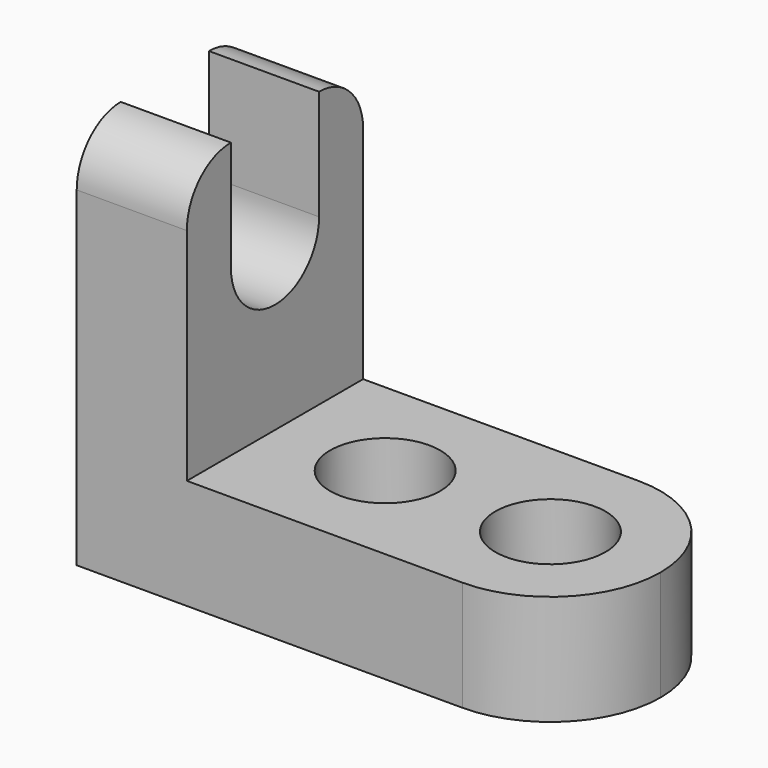
from build123d import *

# Parameters (mm, degrees)
F0_W      = 57.15
F0_H      = 12.7
F1_DEPTH  = 25.4
F2_W      = 12.7
F2_H      = 25.4
F3_DEPTH  = 31.75
F4_R      = 6.35
F5_DEPTH  = 12.701
F7_DEPTH  = 25.4
F9_DEPTH  = 12.701
F10_DEPTH = 25.4
F12_DEPTH = 12.701


# Not quite as in the source:
# - ends of sketch curves that miss each other by under 0.0002 mm in the source are joined


with BuildPart() as f1:
    # F0 (on Front) → F1 (new body)
    with BuildSketch(Plane.XZ):
        with Locations((-32.142091, 22.023173)):
            Rectangle(F0_W, F0_H)
    extrude(amount=F1_DEPTH)

    # F2 (on face) → F3 (join)
    with BuildSketch(Plane.XY.offset(28.373173)):
        with Locations((-54.367091, -12.7)):
            Rectangle(F2_W, F2_H)
    extrude(amount=F3_DEPTH)

    # F4 (on face) → F5 (cut, through all)
    with BuildSketch(Plane.XY.offset(28.373173)):
        with Locations((-16.267091, -12.7)):
            Circle(F4_R)
        with Locations((-35.317091, -12.700001)):
            Circle(F4_R)
    extrude(amount=-F5_DEPTH, mode=Mode.SUBTRACT)

    # F6 (on face) → F7 (cut)
    with BuildSketch(Plane.XY.offset(28.373173)):
        with BuildLine():
            Line((-3.567091, -25.4), (-3.567091, -12.7))
            ThreePointArc((-3.567091, -12.7), (-7.286835, -21.680257), (-16.267091, -25.4))
            Line((-16.267091, -25.4), (-3.567091, -25.4))
        make_face()
        with BuildLine():
            ThreePointArc((-16.267091, 0), (-7.286835, -3.719744), (-3.567091, -12.7))
            Line((-3.567091, -12.7), (-3.567091, 0))
            Line((-3.567091, 0), (-16.267091, 0))
        make_face()
    extrude(amount=-F7_DEPTH, mode=Mode.SUBTRACT)

    # F8 (on face) → F9 (cut, through all)
    with BuildSketch(Plane.YZ.offset(-48.017091)):
        with BuildLine():
            Line((-6.35, 60.123173), (-19.05, 60.123173))
            Line((-19.05, 60.123173), (-19.05, 47.423173))
            ThreePointArc((-19.05, 47.423173), (-12.7, 53.773173), (-6.35, 47.423173))
            Line((-6.35, 47.423173), (-6.35, 60.123173))
        make_face()
        with BuildLine():
            ThreePointArc((-6.35, 47.423173), (-12.7, 53.773173), (-19.05, 47.423173))
            Line((-19.05, 47.423173), (-6.35, 47.423173))
        make_face()
        with BuildLine():
            Line((-6.35, 47.423173), (-19.05, 47.423173))
            ThreePointArc((-19.05, 47.423173), (-12.7, 41.073173), (-6.35, 47.423173))
        make_face()
    extrude(amount=-F9_DEPTH, mode=Mode.SUBTRACT)

    # F10 (cut): a face of the model
    f10_faces = [f1.faces().sort_by_distance(p)[0] for p in [
        (-48.017091, -12.7, 28.779772),
    ]]
    extrude(f10_faces, amount=F10_DEPTH, mode=Mode.SUBTRACT)

    # F11 (on face) → F12 (cut, through all)
    with BuildSketch(Plane.YZ.offset(-48.017091)):
        with BuildLine():
            Line((-19.05, 60.123173), (-25.4, 60.123173))
            Line((-25.4, 60.123173), (-25.4, 53.773173))
            ThreePointArc((-25.4, 53.773173), (-23.540128, 58.263301), (-19.05, 60.123173))
        make_face()
        with BuildLine():
            ThreePointArc((-6.35, 60.123173), (-1.859872, 58.263301), (0, 53.773173))
            Line((0, 53.773173), (0, 60.123173))
            Line((0, 60.123173), (-6.35, 60.123173))
        make_face()
    extrude(amount=-F12_DEPTH, mode=Mode.SUBTRACT)


solid = f1.part
